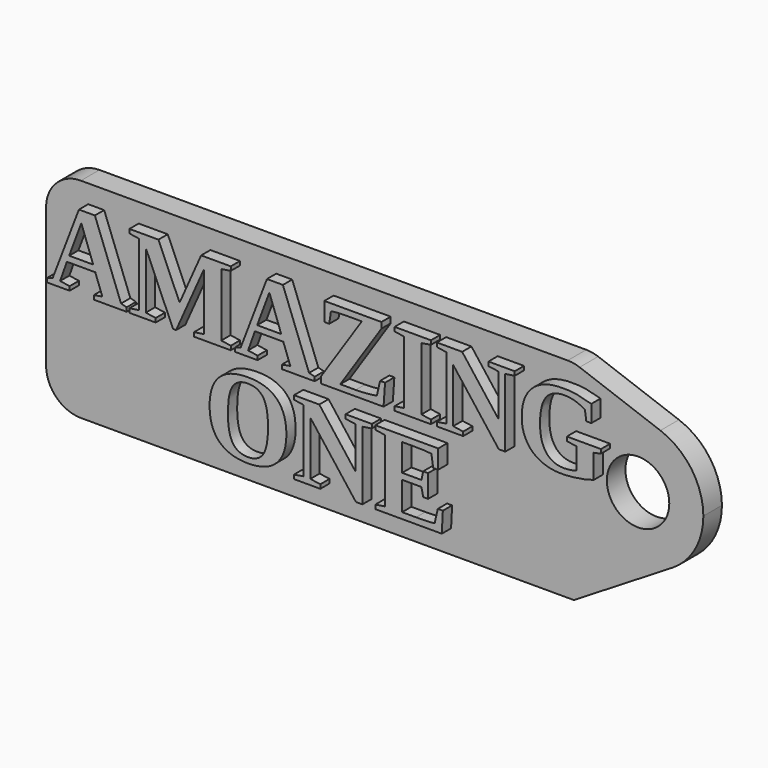
from build123d import *

# Parameters (mm, degrees)
F0_TEXT_SIZE = 9.7222222222
F1_DEPTH     = 1
F2_TEXT_SIZE = 9.7222222222
F3_DEPTH     = 1
F4_R         = 2.69
F5_DEPTH     = 2
F6_DEPTH     = 1
F7_R         = 3


# Not quite as in the source:
# - a feature names something its author has since deleted; it is built from what else it names
# - Text() gives the source's letters only with a copy of the font that has no kerning and outlines rounded to 1/6400 em; it was checked with that copy


with BuildPart() as f1:
    # F0 (on Front) → F1 (new body)
    with BuildSketch(Plane.XZ):
        with Locations((-24.2068142361, -7)):
            Text('AMAZING', F0_TEXT_SIZE, font='Tinos', font_style=FontStyle.BOLD, text_align=(TextAlign.LEFT, TextAlign.BOTTOM))
    extrude(amount=F1_DEPTH)


with BuildPart() as f3:
    # F2 (on Front) → F3 (new body, through all)
    with BuildSketch(Plane.XZ):
        with Locations((-10.5888671875, -15)):
            Text('ONE', F2_TEXT_SIZE, font='Tinos', font_style=FontStyle.BOLD, text_align=(TextAlign.LEFT, TextAlign.BOTTOM))
    extrude(amount=F3_DEPTH)


with BuildPart() as f5:
    # F4 (on Front) → F5 (new body)
    with BuildSketch(Plane.XZ):
        with BuildLine():
            Line((20.4665803953, 1), (-25, 1))
            Line((-25, 1), (-25, -17))
            Line((-25, -17), (20.4665803953, -17))
            Line((20.4665803953, -17), (28.9439704785, -11.7930848961))
            ThreePointArc((28.9439704785, -11.7930848961), (20.4035917374, -7.5664270103), (27.9238633062, -1.7142290081))
            Line((27.9238633062, -1.7142290081), (20.4665803953, 1))
        make_face()
        with BuildLine():
            ThreePointArc((31.625, -7), (30.6077302491, -3.7736325455), (27.9238633062, -1.7142290081))
            ThreePointArc((27.9238633062, -1.7142290081), (20.4035917374, -7.5664270103), (28.9439704785, -11.7930848961))
            ThreePointArc((28.9439704785, -11.7930848961), (30.909198455, -9.7459780642), (31.625, -7))
        make_face()
        with Locations((26, -7)):
            Circle(F4_R, mode=Mode.SUBTRACT)
    extrude(amount=-F5_DEPTH)

    # F7
    f7_edges = [f5.edges().sort_by_distance(p)[0] for p in [
        (-25, 1, 1),
        (20.46658, 1, 1),
        (-25, 1, -17),
    ]]
    fillet(f7_edges, radius=F7_R)


with BuildPart() as f6:
    # F0 (on Front) → F6 (new body, through all)
    with BuildSketch(Plane.XZ):
        with Locations((-24.2068142361, -7)):
            Text('AMAZING', F0_TEXT_SIZE, font='Tinos', font_style=FontStyle.BOLD, text_align=(TextAlign.LEFT, TextAlign.BOTTOM))
    extrude(amount=F6_DEPTH)


solid = Compound([f1.part, f3.part, f5.part, f6.part])
